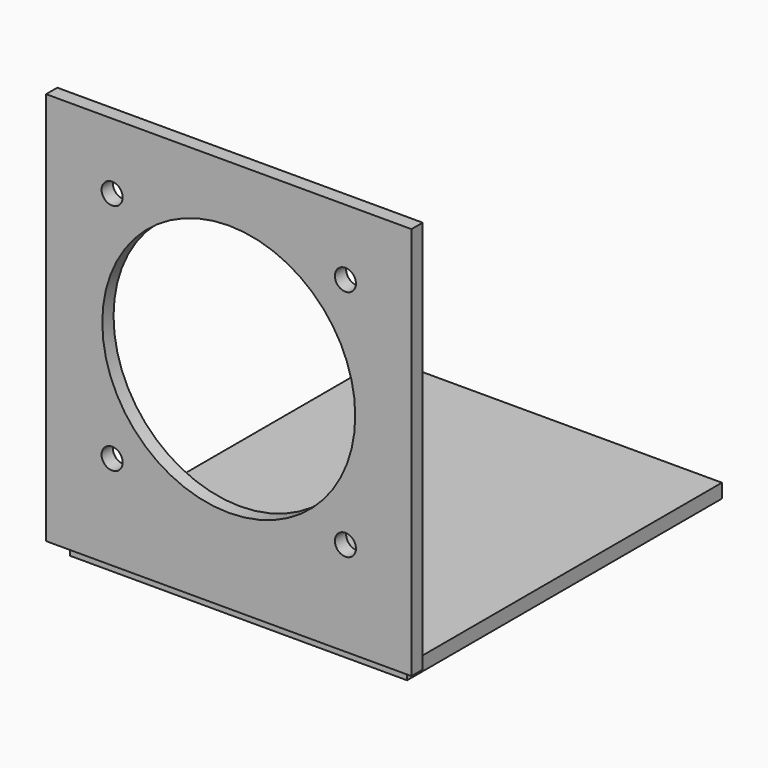
from build123d import *

# Parameters (mm, degrees)
F0_R     = 4.7625
F0_R_2   = 57.15
F1_DEPTH = 6.35
F3_DEPTH = 6.35
F4_W     = 152.4
F4_H     = 6.35
F5_DEPTH = 177.8


# Not quite as in the source:
# - a feature names something its author has since deleted; it is built from what else it names


with BuildPart() as f1:
    # F0 (on Front) → F1 (new body)
    with BuildSketch(Plane.XZ):
        Polygon((82.55, -88.9), (82.55, 88.9), (-82.55, 88.9), (-82.55, -76.2), (-82.55, -88.9), align=None)
        with Locations((-52.705, -46.355)):
            Circle(F0_R, mode=Mode.SUBTRACT)
        with Locations((52.705, -46.355)):
            Circle(F0_R, mode=Mode.SUBTRACT)
        with Locations((-52.705, 59.055)):
            Circle(F0_R, mode=Mode.SUBTRACT)
        with Locations((0, 6.35)):
            Circle(F0_R_2, mode=Mode.SUBTRACT)
        with Locations((52.705, 59.055)):
            Circle(F0_R, mode=Mode.SUBTRACT)
    extrude(amount=F1_DEPTH)

    # F0 (on Front) → F3 (join)
    with BuildSketch(Plane.XZ):
        Polygon((82.55, -88.9), (82.55, 88.9), (-82.55, 88.9), (-82.55, -76.2), (-82.55, -88.9), align=None)
        with Locations((-52.705, -46.355)):
            Circle(F0_R, mode=Mode.SUBTRACT)
        with Locations((52.705, -46.355)):
            Circle(F0_R, mode=Mode.SUBTRACT)
        with Locations((-52.705, 59.055)):
            Circle(F0_R, mode=Mode.SUBTRACT)
        with Locations((0, 6.35)):
            Circle(F0_R_2, mode=Mode.SUBTRACT)
        with Locations((52.705, 59.055)):
            Circle(F0_R, mode=Mode.SUBTRACT)
    extrude(amount=F3_DEPTH)


with BuildPart() as f5:
    # F4 (on face) → F5 (new body)
    with BuildSketch(Plane.XZ.offset(6.35)):
        with Locations((-0.6874045253, -114.6309652448)):
            Rectangle(F4_W, F4_H)
    extrude(amount=-F5_DEPTH)


with BuildPart() as f5_1:
    # F6: moved
    add(f5.part.moved(Location((0, 6.35, 22.352))))


solid = Compound([f1.part, f5_1.part])
